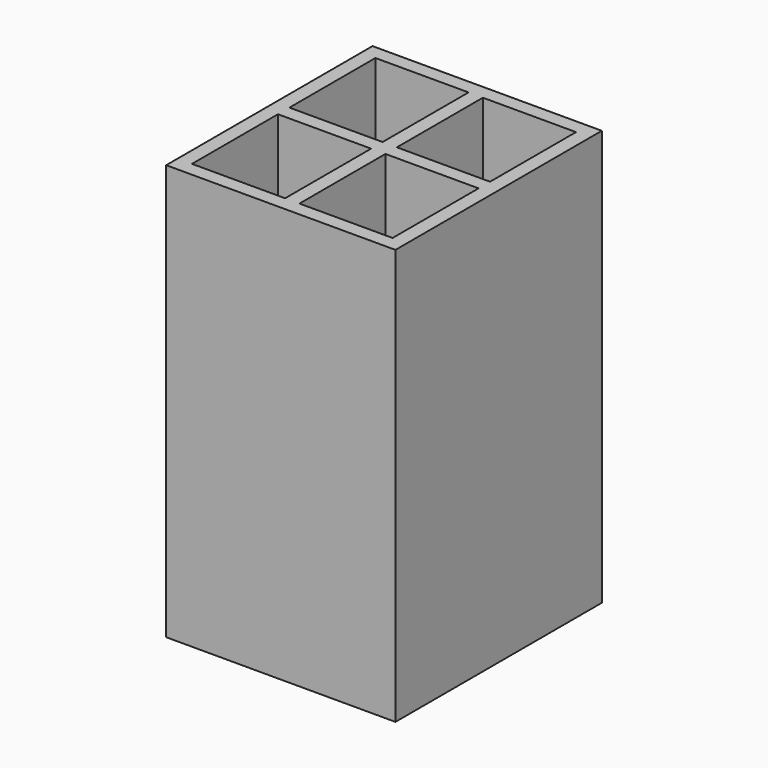
from build123d import *

# Parameters (mm, degrees)
F0_W      = 50.8
F0_H      = 57.15
F1_DEPTH  = 3.175
F2_W      = 50.8
F2_H      = 3.175
F3_DEPTH  = 88.9
F4_W      = 50.8
F4_H      = 3.175
F5_DEPTH  = 88.9
F6_W      = 50.8
F6_H      = 88.9
F7_DEPTH  = 3.175
F8_W      = 57.15
F8_H      = 92.075
F9_DEPTH  = 3.175
F11_W     = 44.45
F11_H     = 3.175
F12_DEPTH = 88.9
F10_W     = 3.175
F10_H     = 50.8
F13_DEPTH = 88.9


with BuildPart() as f1:
    # F0 (on Top) → F1 (new body)
    with BuildSketch(Plane.XY):
        Rectangle(F0_W, F0_H)
    extrude(amount=F1_DEPTH)

    # F2 (on face) → F3 (join)
    with BuildSketch(Plane.XY.offset(3.175)):
        with Locations((0, 26.9875)):
            Rectangle(F2_W, F2_H)
    extrude(amount=F3_DEPTH)

    # F4 (on face) → F5 (join)
    with BuildSketch(Plane.XY.offset(3.175)):
        with Locations((0, -26.9875)):
            Rectangle(F4_W, F4_H)
    extrude(amount=F5_DEPTH)

    # F6 (on face) → F7 (join)
    with BuildSketch(Plane(origin=(-25.4, 0, 0), x_dir=(0, -1, 0), z_dir=(-1, 0, 0))):
        with Locations((0, 47.625)):
            Rectangle(F6_W, F6_H)
    extrude(amount=-F7_DEPTH)

    # F8 (on face) → F9 (join)
    with BuildSketch(Plane.YZ.offset(25.4)):
        with Locations((0, 46.0375)):
            Rectangle(F8_W, F8_H)
    extrude(amount=-F9_DEPTH)

    # F11 (on face) → F12 (join)
    with BuildSketch(Plane.XY.offset(3.175)):
        Rectangle(F11_W, F11_H)
    extrude(amount=F12_DEPTH)

    # F10 (on face) → F13 (join)
    with BuildSketch(Plane.XY.offset(3.175)):
        Rectangle(F10_W, F10_H)
    extrude(amount=F13_DEPTH)


solid = f1.part
